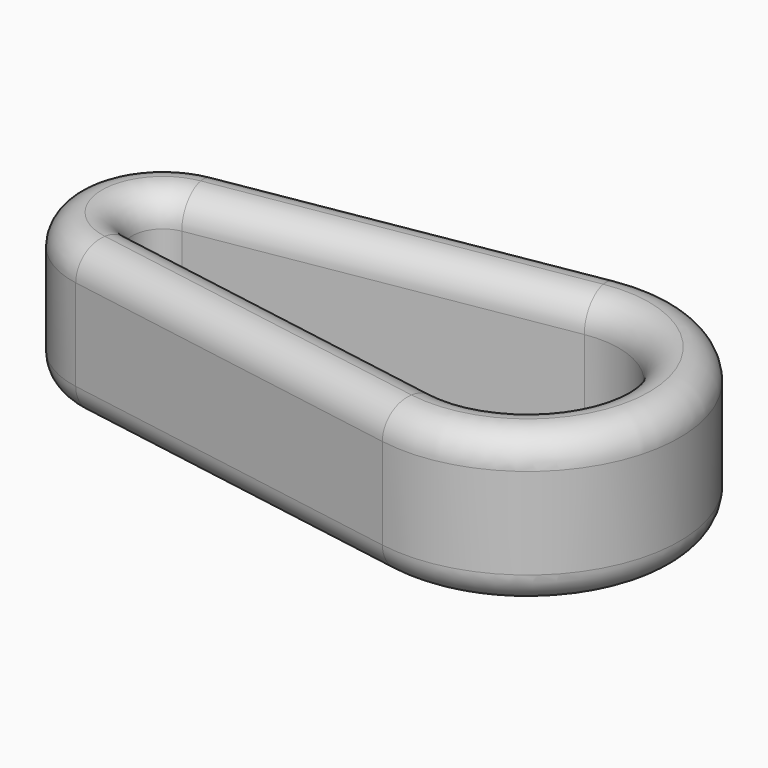
from build123d import *

# Parameters (mm, degrees)
F1_DEPTH = 25
F2_R     = 4.99999


# Not quite as in the source:
# - a fillet or chamfer is up to 0.001 mm smaller than in the source, because OpenCascade refuses the exact size


with BuildPart() as f1:
    # F0 (on Top) → F1 (new body)
    with BuildSketch(Plane.XY):
        with BuildLine():
            Line((-4.1666666667, 24.6503324296), (-62.5, 14.7901994577))
            ThreePointArc((-62.5, 14.7901994577), (-75, 0), (-62.5, -14.7901994577))
            Line((-62.5, -14.7901994577), (-4.1666666667, -24.6503324296))
            ThreePointArc((-4.1666666667, -24.6503324296), (25, 0), (-4.1666666667, 24.6503324296))
        make_face()
        with BuildLine():
            ThreePointArc((-60.8333333333, -4.9300664859), (-65, 0), (-60.8333333333, 4.9300664859))
            Line((-60.8333333333, 4.9300664859), (-2.5, 14.7901994577))
            ThreePointArc((-2.5, 14.7901994577), (15, 0), (-2.5, -14.7901994577))
            Line((-2.5, -14.7901994577), (-60.8333333333, -4.9300664859))
        make_face(mode=Mode.SUBTRACT)
    extrude(amount=F1_DEPTH)

    # F2 (radius 5 in the source; OpenCascade refuses exactly that, so slightly less here)
    f2_edges = [f1.edges().sort_by_distance(p)[0] for p in [
        (25, 0, 25),
        (-33.333333, 19.720266, 25),
        (-75, 0, 25),
        (-33.333333, -19.720266, 25),
        (-31.666667, 9.860133, 25),
        (15, 0, 25),
        (-31.666667, -9.860133, 25),
        (-65, 0, 25),
        (-4.166667, -24.650332, 12.5),
        (-4.166667, 24.650332, 12.5),
        (25, 0, 0),
    ]]
    fillet(f2_edges, radius=F2_R)


solid = f1.part
